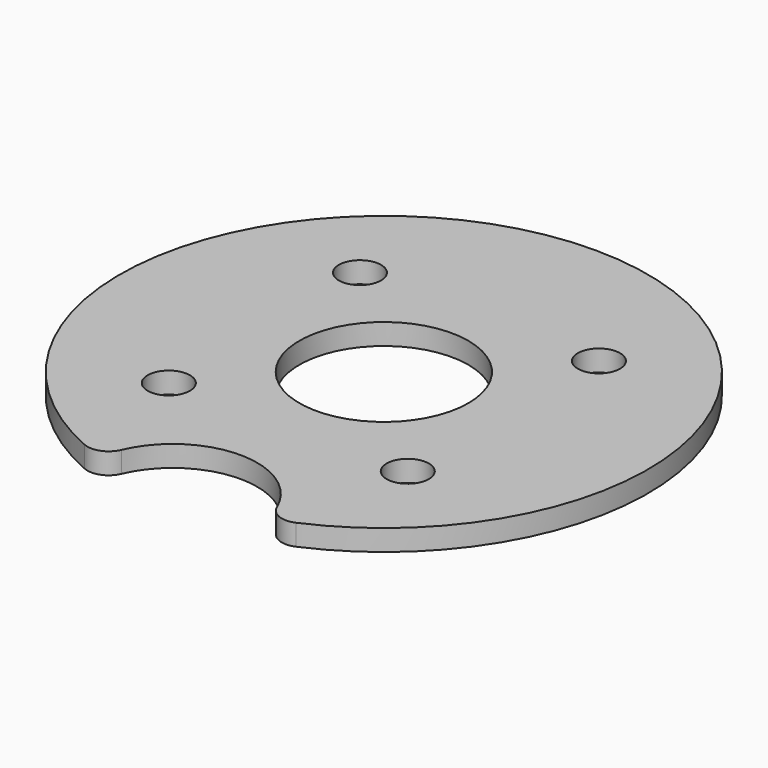
from build123d import *

# Parameters (mm, degrees)
F0_R     = 12.5
F0_R_2   = 1
F0_R_3   = 4
F2_R     = 4
F4_DEPTH = 1
F5_R     = 1


with BuildPart() as f3:
    # F3: sweep along a path in F1
    with BuildLine(Plane.XZ) as f3_path:
        Line((0, 0), (0, 1))
    # F0 (on Top) → F3 (sweep)
    with BuildSketch(Plane.XY):
        Circle(F0_R)
        with Locations((-5.6568542495, -5.6568542495)):
            Circle(F0_R_2, mode=Mode.SUBTRACT)
        with Locations((5.6568542495, -5.6568542495)):
            Circle(F0_R_2, mode=Mode.SUBTRACT)
        with Locations((-5.6568542495, 5.6568542495)):
            Circle(F0_R_2, mode=Mode.SUBTRACT)
        Circle(F0_R_3, mode=Mode.SUBTRACT)
        with Locations((5.6568542495, 5.6568542495)):
            Circle(F0_R_2, mode=Mode.SUBTRACT)
    sweep(path=f3_path.line)

    # F2 (on Top) → F4 (cut, through all)
    with BuildSketch(Plane.XY):
        with Locations((0, -12.5)):
            Circle(F2_R)
    extrude(amount=F4_DEPTH, mode=Mode.SUBTRACT)

    # F5
    f5_edges = [f3.edges().sort_by_distance(p)[0] for p in [
        (-3.948468, -11.86, 0.5),
        (3.948468, -11.86, 0.5),
    ]]
    fillet(f5_edges, radius=F5_R)


solid = f3.part
